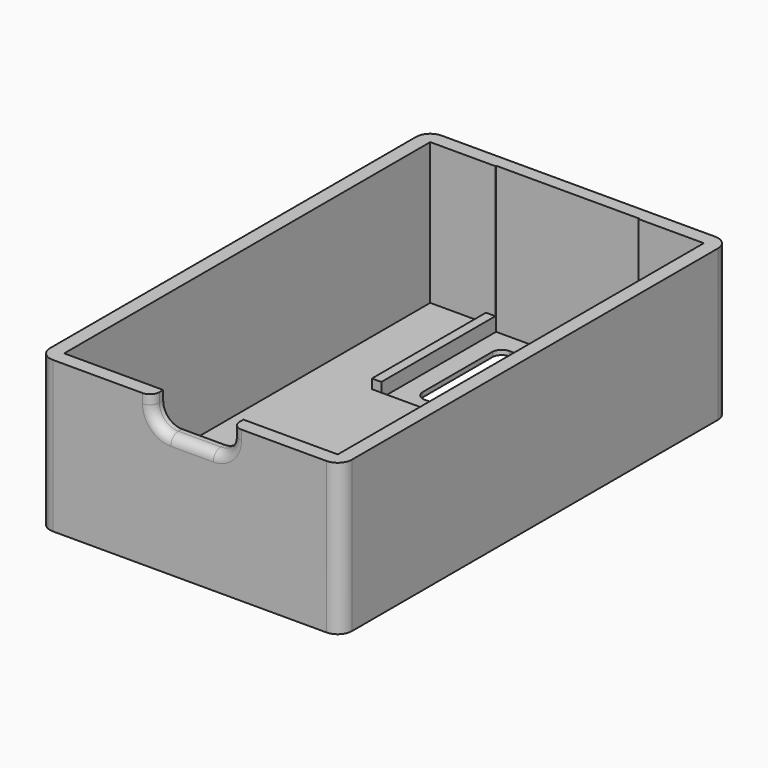
from build123d import *

# Parameters (mm, degrees)
F0_W      = 32
F0_H      = 51.5
F1_DEPTH  = 1
F2_DEPTH  = 16
F3_R      = 1.5
F4_W      = 8.5
F4_H      = 3
F5_DEPTH  = 5
F6_R      = 2
F7_R      = 1
F0_W_2    = 15.2
F0_H_2    = 13.6
F0_W_3    = 11.1999999404
F0_H_3    = 11.1999999404
F0_H_4    = 0.1
F0_H_5    = 1.5
F8_DEPTH  = 0.5
F9_R      = 1
F10_W     = 1
F10_H     = 15.1
F11_DEPTH = 1


with BuildPart() as f1:
    # F0 (on Top) → F1 (new body)
    with BuildSketch(Plane.XY):
        Rectangle(F0_W, F0_H)
        Polygon((7.6, 24.35), (7.6, 24.25), (14.5, 24.25), (14.5, -24.25), (-14.5, -24.25), (-14.5, 24.25), (-7.6, 24.25), (-7.6, 24.35), align=None, mode=Mode.SUBTRACT)
        Polygon((13, 22.75), (13, -22.75), (-13, -22.75), (-13, 22.75), (-7.6, 22.75), (-7.6, 24.25), (-14.5, 24.25), (-14.5, -24.25), (14.5, -24.25), (14.5, 24.25), (7.6, 24.25), (7.6, 22.75), align=None)
        Polygon((-13, -22.75), (13, -22.75), (13, 22.75), (7.6, 22.75), (7.6, 9.15), (-7.6, 9.15), (-7.6, 22.75), (-13, 22.75), align=None)
    extrude(amount=F1_DEPTH)

    # F0 (on Top) → F2 (join)
    with BuildSketch(Plane.XY):
        Rectangle(F0_W, F0_H)
        Polygon((7.6, 24.35), (7.6, 24.25), (14.5, 24.25), (14.5, -24.25), (-14.5, -24.25), (-14.5, 24.25), (-7.6, 24.25), (-7.6, 24.35), align=None, mode=Mode.SUBTRACT)
    extrude(amount=F2_DEPTH)

    # F3
    f3_edges = [f1.edges().sort_by_distance(p)[0] for p in [
        (-16, -25.75, 8),
        (16, -25.75, 8),
        (-16, 25.75, 8),
        (16, 25.75, 8),
    ]]
    fillet(f3_edges, radius=F3_R)

    # F4 (on face) → F5 (cut)
    with BuildSketch(Plane.XZ.offset(25.75)):
        with Locations((0.25, 14.5)):
            Rectangle(F4_W, F4_H)
    extrude(amount=-F5_DEPTH, mode=Mode.SUBTRACT)

    # F6
    f6_edges = [f1.edges().sort_by_distance(p)[0] for p in [
        (-4, -25, 13),
        (4.5, -25, 13),
    ]]
    fillet(f6_edges, radius=F6_R)

    # F7
    f7_edges = [f1.edges().sort_by_distance(p)[0] for p in [
        (-3.414214, -25.75, 13.585786),
        (0.25, -25.75, 13),
    ]]
    fillet(f7_edges, radius=F7_R)

    # F0 (on Top) → F8 (join)
    with BuildSketch(Plane.XY):
        with Locations((0, 15.95)):
            Rectangle(F0_W_2, F0_H_2)
        with Locations((0, 16.75)):
            Rectangle(F0_W_3, F0_H_3, mode=Mode.SUBTRACT)
        with Locations((0, 24.3)):
            Rectangle(F0_W_2, F0_H_4)
        with Locations((0, 23.5)):
            Rectangle(F0_W_2, F0_H_5)
    extrude(amount=F8_DEPTH)

    # F9
    f9_edges = [f1.edges().sort_by_distance(p)[0] for p in [
        (5.6, 11.15, 0.25),
        (-5.6, 11.15, 0.25),
        (5.6, 22.35, 0.25),
        (-5.6, 22.35, 0.25),
    ]]
    fillet(f9_edges, radius=F9_R)

    # F10 (on face) → F11 (join)
    with BuildSketch(Plane.XY.offset(1)):
        with Locations((-8.1, 16.7)):
            Rectangle(F10_W, F10_H)
        with Locations((8.1, 16.7)):
            Rectangle(F10_W, F10_H)
    extrude(amount=F11_DEPTH)


solid = f1.part
